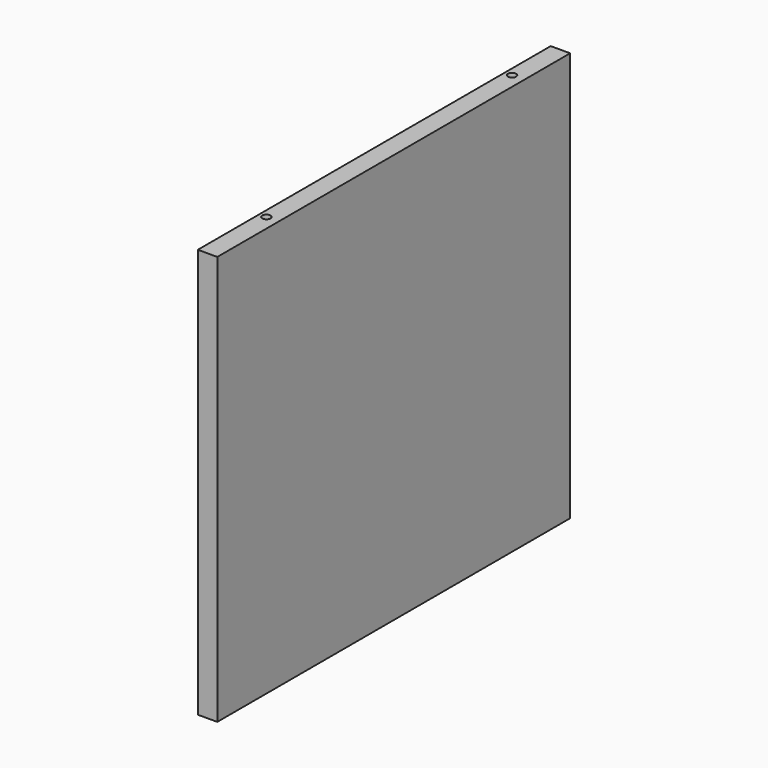
from build123d import *

# Parameters (mm, degrees)
F0_W     = 431
F0_H     = 400
F1_DEPTH = 19
F2_R     = 12.5
F3_DEPTH = 12
F5_D     = 8
F5_DEPTH = 22
F5_TIP   = 2.4034424761


# Not quite as in the source:
# - a pattern or mirror of a feature is missing from the dataset's text; its kind, count and spacing are read off the source's solid


with BuildPart() as f1:
    # F0 (on Right) → F1 (new body)
    with BuildSketch(Plane.YZ):
        Rectangle(F0_W, F0_H)
    extrude(amount=F1_DEPTH)

    # F2 (on face) → F3 (cut)
    with BuildSketch(Plane(origin=(0, 0, 0), x_dir=(0, -1, 0), z_dir=(-1, 0, 0))):
        with Locations((-159.5, 166.5)):
            Circle(F2_R)
        with Locations((140.5, 166.5)):
            Circle(F2_R)
        with Locations((140.5, -166.5)):
            Circle(F2_R)
        with Locations((-159.5, -166.5)):
            Circle(F2_R)
    extrude(amount=-F3_DEPTH, mode=Mode.SUBTRACT)

    # F5
    with Locations(Plane.XY.offset(200)):
        with Locations((7, 159.5), (7, -140.5)):
            f5 = Hole(F5_D / 2, depth=F5_DEPTH)
            with Locations((0, 0, -(F5_DEPTH + F5_TIP / 2))):  # 118° drill point
                Cone(0, F5_D / 2, F5_TIP, mode=Mode.SUBTRACT)

    # F5_copies: F5 across plane
    add(f5.mirror(Plane(origin=(0, 0, 2.1e-05), x_dir=(-1, 0, 0), z_dir=(0, 0, -1))), mode=Mode.SUBTRACT)


solid = f1.part
